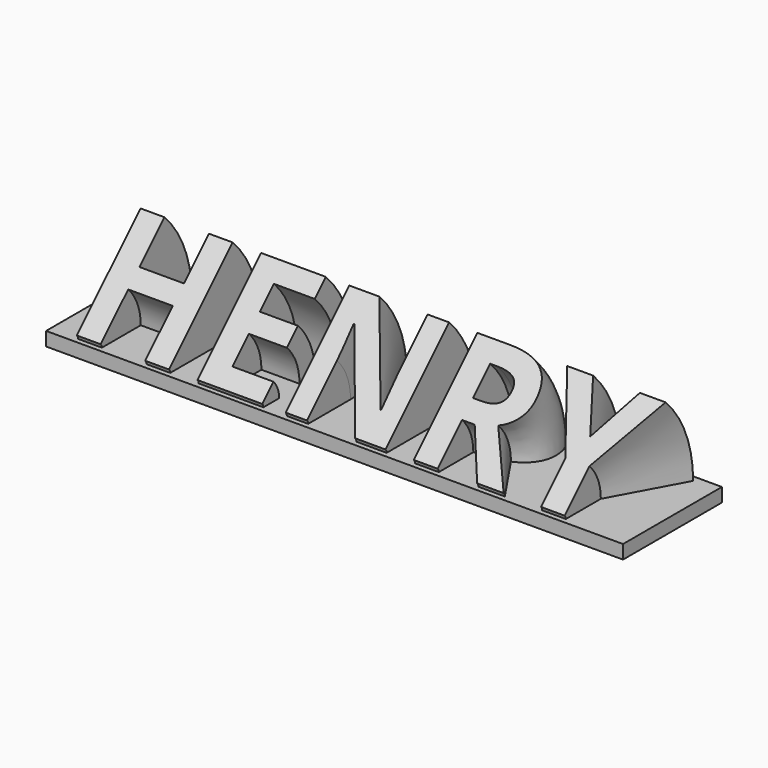
from build123d import *

# Parameters (mm, degrees)
F0_W         = 53.34
F0_H         = 11.43
F0_TEXT_SIZE = 14.5676135854
F1_DEPTH     = 1.27
F2_ANGLE     = 45


# Not quite as in the source:
# - Text() gives the source's letters only with a copy of the font that has no kerning and outlines rounded to 1/6400 em; it was checked with that copy


with BuildPart() as f1:
    # F0 (on Top) → F1 (new body)
    with BuildSketch(Plane.XY):
        Rectangle(F0_W, F0_H)
        Polygon((-15.5691370194, 5.1555694955), (-15.5691370194, -5.2443408908), (-17.767936195, -5.2443408908), (-17.767936195, -0.7556949547), (-21.8855632225, -0.7556949547), (-21.8855632225, -5.2443408908), (-24.0911909669, -5.2443408908), (-24.0911909669, 5.1555694955), (-21.8855632225, 5.1555694955), (-21.8855632225, 1.0789138812), (-17.767936195, 1.0789138812), (-17.767936195, 5.1555694955), align=None, mode=Mode.SUBTRACT)
        Polygon((-6.9560354871, -3.4233891926), (-6.9560354871, -5.2443408908), (-12.9446903844, -5.2443408908), (-12.9446903844, 5.1555694955), (-6.9560354871, 5.1555694955), (-6.9560354871, 3.348274935), (-10.73906264, 3.348274935), (-10.73906264, 1.0652567434), (-7.2177972937, 1.0652567434), (-7.2177972937, -0.742037817), (-10.73906264, -0.742037817), (-10.73906264, -3.4233891926), align=None, mode=Mode.SUBTRACT)
        with BuildLine():
            Line((4.4385697643, 5.1555694955), (4.4385697643, -5.2443408908))
            Line((4.4385697643, -5.2443408908), (1.6365803387, -5.2443408908))
            Line((1.6365803387, -5.2443408908), (-2.8884846312, 2.6221704454))
            Line((-2.8884846312, 2.6221704454), (-2.9522179407, 2.6221704454))
            add(Edge.make_bspline(
                [(-2.9522179407, 2.6221704454), (-2.8156465633, 0.5394569406), (-2.8156465633, -0.3505332019)],
                knots=[0, 0, 0, 1, 1, 1], degree=2))
            Line((-2.8156465633, -0.3505332019), (-2.8156465633, -5.2443408908))
            Line((-2.8156465633, -5.2443408908), (-4.7868267766, -5.2443408908))
            Line((-4.7868267766, -5.2443408908), (-4.7868267766, 5.1555694955))
            Line((-4.7868267766, 5.1555694955), (-2.0053230576, 5.1555694955))
            Line((-2.0053230576, 5.1555694955), (2.5106371539, -2.6335513935))
            Line((2.5106371539, -2.6335513935), (2.5607133256, -2.6335513935))
            add(Edge.make_bspline(
                [(2.5607133256, -2.6335513935), (2.4537324133, -0.6054664396), (2.4537324133, 0.2321713415)],
                knots=[0, 0, 0, 1, 1, 1], degree=2))
            Line((2.4537324133, 0.2321713415), (2.4537324133, 5.1555694955))
            Line((2.4537324133, 5.1555694955), (4.4385697643, 5.1555694955))
        make_face(mode=Mode.SUBTRACT)
        with BuildLine():
            Line((10.4340532306, -1.2541804821), (9.2618155749, -1.2541804821))
            Line((9.2618155749, -1.2541804821), (9.2618155749, -5.2443408908))
            Line((9.2618155749, -5.2443408908), (7.0561878305, -5.2443408908))
            Line((7.0561878305, -5.2443408908), (7.0561878305, 5.1555694955))
            Line((7.0561878305, 5.1555694955), (10.0857962183, 5.1555694955))
            add(Edge.make_bspline(
                [(10.0857962183, 5.1555694955), (12.2072049467, 5.1555694955), (13.2235236132, 4.3839412134)],
                knots=[0, 0, 0, 1, 1, 1], degree=2))
            add(Edge.make_bspline(
                [(13.2235236132, 4.3839412134), (14.2398422798, 3.6123129313), (14.2398422798, 2.039465902)],
                knots=[0, 0, 0, 1, 1, 1], degree=2))
            add(Edge.make_bspline(
                [(14.2398422798, 2.039465902), (14.2398422798, 1.122161484), (13.7356662783, 0.4074379425)],
                knots=[0, 0, 0, 1, 1, 1], degree=2))
            add(Edge.make_bspline(
                [(13.7356662783, 0.4074379425), (13.2314902769, -0.3072855991), (12.3050811005, -0.7124473519)],
                knots=[0, 0, 0, 1, 1, 1], degree=2))
            add(Edge.make_bspline(
                [(12.3050811005, -0.7124473519), (14.6541087911, -4.2200555605), (15.3642799534, -5.2443408908)],
                knots=[0, 0, 0, 1, 1, 1], degree=2))
            Line((15.3642799534, -5.2443408908), (12.917376109, -5.2443408908))
            Line((12.917376109, -5.2443408908), (10.4340532306, -1.2541804821))
        make_face(mode=Mode.SUBTRACT)
        Polygon((17.7542790573, 5.1555694955), (19.90983063, 0.8740568151), (22.0790393404, 5.1555694955), (24.4553813066, 5.1555694955), (21.0046778385, -1.1972757416), (21.0046778385, -5.2443408908), (18.8149834215, -5.2443408908), (18.8149834215, -1.2678376199), (15.3642799534, 5.1555694955), align=None, mode=Mode.SUBTRACT)
        with BuildLine():
            Line((9.2618155749, 3.348274935), (9.2618155749, 0.5394569406))
            Line((9.2618155749, 0.5394569406), (9.9719867372, 0.5394569406))
            add(Edge.make_bspline(
                [(9.9719867372, 0.5394569406), (11.0190339636, 0.5394569406), (11.5163813962, 0.8877139529)],
                knots=[0, 0, 0, 1, 1, 1], degree=2))
            add(Edge.make_bspline(
                [(11.5163813962, 0.8877139529), (12.0137288287, 1.2359709651), (12.0137288287, 1.9825611614)],
                knots=[0, 0, 0, 1, 1, 1], degree=2))
            add(Edge.make_bspline(
                [(12.0137288287, 1.9825611614), (12.0137288287, 2.7223227888), (11.5050004481, 3.0352988619)],
                knots=[0, 0, 0, 1, 1, 1], degree=2))
            add(Edge.make_bspline(
                [(11.5050004481, 3.0352988619), (10.9962720674, 3.348274935), (9.931015324, 3.348274935)],
                knots=[0, 0, 0, 1, 1, 1], degree=2))
            Line((9.931015324, 3.348274935), (9.2618155749, 3.348274935))
        make_face()
        with Locations((-25.4, -5.2443408908)):
            Text('HENRY', F0_TEXT_SIZE, font='Open Sans', font_style=FontStyle.BOLD, text_align=(TextAlign.LEFT, TextAlign.BOTTOM))
    extrude(amount=-F1_DEPTH)

    # F0 (on Top) → F2 (revolve)
    with BuildSketch(Plane.XY):
        with Locations((-25.4, -5.2443408908)):
            Text('HENRY', F0_TEXT_SIZE, font='Open Sans', font_style=FontStyle.BOLD, text_align=(TextAlign.LEFT, TextAlign.BOTTOM))
    revolve(axis=Axis((0, -5.715, 0), (1, 0, 0)), revolution_arc=F2_ANGLE)


solid = f1.part
